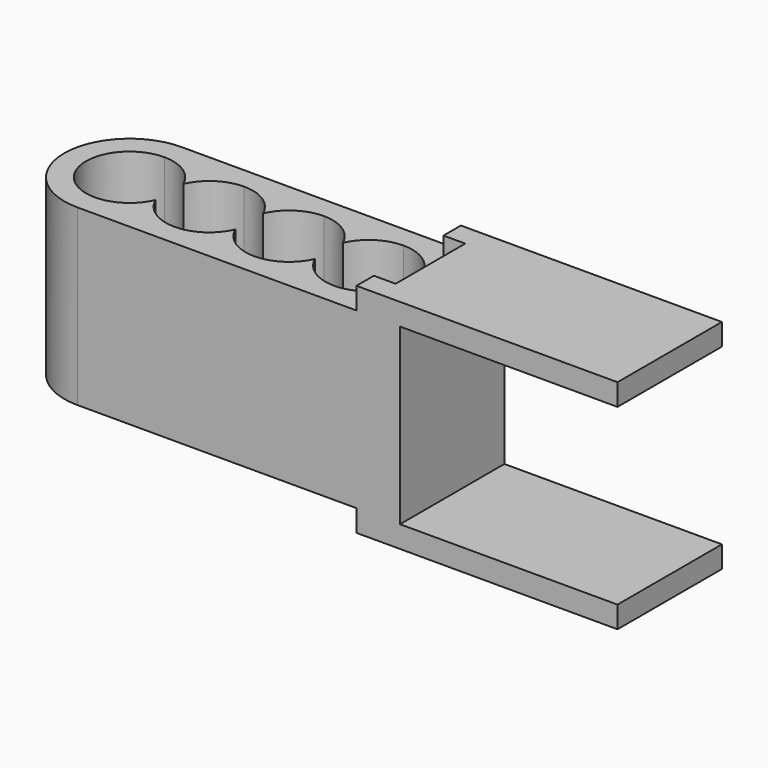
from build123d import *

# Parameters (mm, degrees)
F1_DEPTH    = 12.7
F0_W        = 3.175
F0_H        = 12.7
F0_W_2      = 28.575
F0_H_2      = 3.175
F2_DEPTH    = 15.875
F3_T        = 3.175
F3_T3_DEPTH = 9.525
F3_T5_DEPTH = 9.525
F3_T7_DEPTH = 31.75
F3_T9_DEPTH = 38.1
F4_W        = 3.175
F4_H        = 25.4
F5_DEPTH    = 31.75


# Not quite as in the source:
# - a shell that OpenCascade refuses in one call is made with other operations: the cavity is built on its own and cut out


with BuildPart() as f1:
    # F0 (on Top) → F1 (new body, symmetric)
    with BuildSketch(Plane.XY):
        with BuildLine():
            Line((40.739098, 9.525), (0, 9.525))
            ThreePointArc((0, 9.525), (-9.525, 0), (0, -9.525))
            Line((0, -9.525), (40.739098, -9.525))
            Line((40.739098, -9.525), (40.739098, -6.35))
            Line((40.739098, -6.35), (34.919227, -6.35))
            Line((34.919227, -6.35), (23.279485, -6.35))
            Line((23.279485, -6.35), (11.639742, -6.35))
            Line((11.639742, -6.35), (0, -6.35))
            ThreePointArc((0, -6.35), (-6.35, 0), (0, 6.35))
            Line((0, 6.35), (11.639742, 6.35))
            Line((11.639742, 6.35), (23.279485, 6.35))
            Line((23.279485, 6.35), (34.919227, 6.35))
            Line((34.919227, 6.35), (40.739098, 6.35))
            Line((40.739098, 6.35), (40.739098, 9.525))
        make_face()
        with BuildLine():
            ThreePointArc((5.819871, 2.54), (8.161704, 5.312791), (11.639742, 6.35))
            Line((11.639742, 6.35), (0, 6.35))
            ThreePointArc((0, 6.35), (3.478038, 5.312791), (5.819871, 2.54))
        make_face()
        with BuildLine():
            ThreePointArc((17.459613, 2.54), (19.801446, 5.312791), (23.279485, 6.35))
            Line((23.279485, 6.35), (11.639742, 6.35))
            ThreePointArc((11.639742, 6.35), (15.11778, 5.312791), (17.459613, 2.54))
        make_face()
        with BuildLine():
            ThreePointArc((29.099356, 2.54), (31.441189, 5.312791), (34.919227, 6.35))
            Line((34.919227, 6.35), (23.279485, 6.35))
            ThreePointArc((23.279485, 6.35), (26.757523, 5.312791), (29.099356, 2.54))
        make_face()
        with BuildLine():
            Line((40.739098, 2.54), (40.739098, 6.35))
            Line((40.739098, 6.35), (34.919227, 6.35))
            ThreePointArc((34.919227, 6.35), (38.397265, 5.312791), (40.739098, 2.54))
        make_face()
        with BuildLine():
            Line((23.279485, -6.35), (34.919227, -6.35))
            ThreePointArc((34.919227, -6.35), (31.441189, -5.312791), (29.099356, -2.54))
            ThreePointArc((29.099356, -2.54), (26.757523, -5.312791), (23.279485, -6.35))
        make_face()
        with BuildLine():
            Line((34.919227, -6.35), (40.739098, -6.35))
            Line((40.739098, -6.35), (40.739098, -2.54))
            ThreePointArc((40.739098, -2.54), (38.397265, -5.312791), (34.919227, -6.35))
        make_face()
        with BuildLine():
            Line((11.639742, -6.35), (23.279485, -6.35))
            ThreePointArc((23.279485, -6.35), (19.801446, -5.312791), (17.459613, -2.54))
            ThreePointArc((17.459613, -2.54), (15.117781, -5.312791), (11.639742, -6.35))
        make_face()
        with BuildLine():
            Line((0, -6.35), (11.639742, -6.35))
            ThreePointArc((11.639742, -6.35), (8.161704, -5.312791), (5.819871, -2.54))
            ThreePointArc((5.819871, -2.54), (3.478038, -5.312791), (0, -6.35))
        make_face()
    extrude(amount=F1_DEPTH, both=True)

    # F0 (on Top) → F2 (join, symmetric)
    with BuildSketch(Plane.XY):
        with Locations((45.501598, 0)):
            Rectangle(F0_W, F0_H)
        with Locations((61.376598, 0)):
            Rectangle(F0_W_2, F0_H)
        with Locations((77.251598, 0)):
            Rectangle(F0_W, F0_H)
        with Locations((45.501598, 7.9375)):
            Rectangle(F0_W, F0_H_2)
        with Locations((42.326598, 7.9375)):
            Rectangle(F0_W, F0_H_2)
        with Locations((61.376598, 7.9375)):
            Rectangle(F0_W_2, F0_H_2)
        with Locations((77.251598, 7.9375)):
            Rectangle(F0_W, F0_H_2)
        with Locations((42.326598, -7.9375)):
            Rectangle(F0_W, F0_H_2)
        with Locations((45.501598, -7.9375)):
            Rectangle(F0_W, F0_H_2)
        with Locations((61.376598, -7.9375)):
            Rectangle(F0_W_2, F0_H_2)
        with Locations((77.251598, -7.9375)):
            Rectangle(F0_W, F0_H_2)
    extrude(amount=F2_DEPTH, both=True)

    # F3: shell of thickness 3.175, made by hand


with BuildPart() as f3_core1:
    # F3_t2: copy of F1
    add(f1.part)

    # the walls: a layer under each face that stays
    f3_faces = [f3_core1.faces().sort_by_distance(p)[0] for p in [
        (39.419549, 9.525, 0),
        (-1.14765, -6.35, -12.7),
        (-9.525, 0, 0),
        (-1.14765, -6.35, 12.7),
        (39.419549, -9.525, 0),
        (40.739098, -7.9375, -14.2875),
        (40.739098, -4.445, 0),
        (34.919227, -6.35, 0),
        (23.279485, -6.35, 0),
        (11.639742, -6.35, 0),
        (-6.35, 0, 0),
        (11.639742, 6.35, 0),
        (23.279485, 6.35, 0),
        (34.919227, 6.35, 0),
        (40.739098, 4.445, 0),
        (40.739098, 7.9375, -14.2875),
        (40.739098, -7.9375, 14.2875),
        (40.739098, 7.9375, 14.2875),
        (59.789098, 0, -15.875),
        (59.789098, 0, 15.875),
        (42.326598, -6.35, 0),
        (42.326598, 6.35, 0),
        (43.914098, 0, 0),
    ]]
    thicken(f3_faces, amount=-F3_T, mode=Mode.SUBTRACT)

    # F3_s4 → F3_t3 (cut)
    with BuildSketch(Plane.XZ.offset(3.175)):
        Polygon((40.707348, -12.73175), (40.739098, -9.525), (43.914098, -9.525), (43.914098, -12.7), align=None)
        Polygon((40.707348, 12.73175), (40.739098, 9.525), (43.914098, 9.525), (43.914098, 12.7), align=None)
    extrude(amount=F3_T3_DEPTH, mode=Mode.SUBTRACT)

    # F3_s6 → F3_t5 (cut)
    with BuildSketch(Plane.XZ.offset(-12.7)):
        Polygon((40.707348, -12.73175), (40.739098, -9.525), (43.914098, -9.525), (43.914098, -12.7), align=None)
        Polygon((40.707348, 12.73175), (40.739098, 9.525), (43.914098, 9.525), (43.914098, 12.7), align=None)
    extrude(amount=F3_T5_DEPTH, mode=Mode.SUBTRACT)

    # F3_s8 → F3_t7 (cut)
    with BuildSketch(Plane.XY.offset(-15.875)):
        Polygon((40.770848, -6.31825), (37.564098, -6.35), (37.564098, -9.525), (40.739098, -9.525), align=None)
        Polygon((40.770848, 6.31825), (37.564098, 6.35), (37.564098, 9.525), (40.739098, 9.525), align=None)
    extrude(amount=F3_T7_DEPTH, mode=Mode.SUBTRACT)

    # F3_s10 → F3_t9 (cut)
    with BuildSketch(Plane.XY.offset(-19.05)):
        Polygon((43.882348, -6.31825), (43.914098, -9.525), (47.089098, -9.525), (47.089098, -6.35), align=None)
        Polygon((43.882348, 6.31825), (43.914098, 9.525), (47.089098, 9.525), (47.089098, 6.35), align=None)
    extrude(amount=F3_T9_DEPTH, mode=Mode.SUBTRACT)


with BuildPart() as f1_1:
    add(f1.part)

    # what is left inside the walls is the cavity
    f3_cavity = [f3_core1.part.solids().sort_by_distance(p)[0] for p in [
        (62.964098, 6.31825, -4.233333),
    ]]
    add(f3_cavity, mode=Mode.SUBTRACT)

    # F4 (on face) → F5 (cut, through all)
    with BuildSketch(Plane.YZ.offset(78.839098)):
        with Locations((7.9375, 0)):
            Rectangle(F4_W, F4_H)
        with Locations((-7.9375, 0)):
            Rectangle(F4_W, F4_H)
    extrude(amount=-F5_DEPTH, mode=Mode.SUBTRACT)


solid = f1_1.part
